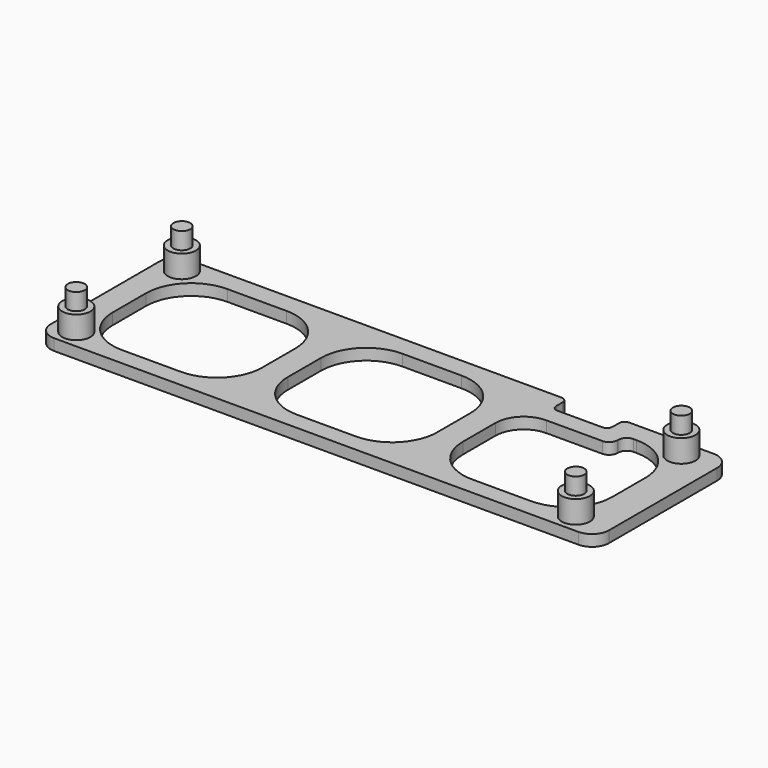
from build123d import *

# Parameters (mm, degrees)
F1_DEPTH = 2
F3_R     = 3
F4_R     = 1
F2_R     = 2.5
F2_R_2   = 1.5
F5_DEPTH = 4
F6_DEPTH = 7


with BuildPart() as f1:
    # F0 (on Top) → F1 (new body)
    with BuildSketch(Plane.XY):
        Polygon((80, -3.433377482), (70, -3.433377482), (70, 0), (0, 0), (0, -30), (99, -30), (99, 0), (80, 0), align=None)
        with BuildLine():
            ThreePointArc((4.5, -11.5), (6.8431457505, -5.8431457505), (12.5, -3.5))
            Line((12.5, -3.5), (23, -3.5))
            ThreePointArc((23, -3.5), (28.6568542495, -5.8431457505), (31, -11.5))
            Line((31, -11.5), (31, -18.9))
            ThreePointArc((31, -18.9), (28.6568542495, -24.5568542495), (23, -26.9))
            Line((23, -26.9), (12.5, -26.9))
            ThreePointArc((12.5, -26.9), (6.8431457505, -24.5568542495), (4.5, -18.9))
            Line((4.5, -18.9), (4.5, -11.5))
        make_face(mode=Mode.SUBTRACT)
        with BuildLine():
            ThreePointArc((35.55, -11.5), (37.8931457505, -5.8431457505), (43.55, -3.5))
            Line((43.55, -3.5), (54.05, -3.5))
            ThreePointArc((54.05, -3.5), (59.7068542495, -5.8431457505), (62.05, -11.5))
            Line((62.05, -11.5), (62.05, -18.9))
            ThreePointArc((62.05, -18.9), (59.7068542495, -24.5568542495), (54.05, -26.9))
            Line((54.05, -26.9), (43.55, -26.9))
            ThreePointArc((43.55, -26.9), (37.8931457505, -24.5568542495), (35.55, -18.9))
            Line((35.55, -18.9), (35.55, -11.5))
        make_face(mode=Mode.SUBTRACT)
        with BuildLine():
            Line((84.5458595753, -3.5), (85.1, -3.5))
            ThreePointArc((85.1, -3.5), (90.7568542495, -5.8431457505), (93.1, -11.5))
            Line((93.1, -11.5), (93.1, -18.9))
            ThreePointArc((93.1, -18.9), (90.7568542495, -24.5568542495), (85.1, -26.9))
            Line((85.1, -26.9), (74.6, -26.9))
            ThreePointArc((74.6, -26.9), (68.9431457505, -24.5568542495), (66.6, -18.9))
            Line((66.6, -18.9), (66.6, -11.6456231289))
            ThreePointArc((66.6, -11.6456231289), (68.0644660941, -8.1100892229), (71.6, -6.6456231289))
            Line((71.6, -6.6456231289), (81.5458595753, -6.6456231289))
            ThreePointArc((81.5458595753, -6.6456231289), (82.6065197471, -6.2062833006), (83.0458595753, -5.1456231289))
            Line((83.0458595753, -5.1456231289), (83.0458595753, -5))
            ThreePointArc((83.0458595753, -5), (83.4851994035, -3.9393398282), (84.5458595753, -3.5))
        make_face(mode=Mode.SUBTRACT)
    extrude(amount=-F1_DEPTH)

    # F3
    f3_edges = [f1.edges().sort_by_distance(p)[0] for p in [
        (0, 0, -1),
        (0, -30, -1),
        (99, -30, -1),
        (99, 0, -1),
    ]]
    fillet(f3_edges, radius=F3_R)

    # F4
    f4_edges = [f1.edges().sort_by_distance(p)[0] for p in [
        (70, -3.433377, -1),
        (80, -3.433377, -1),
        (70, 0, -1),
        (80, 0, -1),
    ]]
    fillet(f4_edges, radius=F4_R)

    # F2 (on face) → F5 (join)
    with BuildSketch(Plane.XY):
        with Locations((4.2, -3.2)):
            Circle(F2_R)
        with Locations((4.2, -3.2)):
            Circle(F2_R_2, mode=Mode.SUBTRACT)
        with Locations((92.8, -3.2)):
            Circle(F2_R)
        with Locations((92.8, -3.2)):
            Circle(F2_R_2, mode=Mode.SUBTRACT)
        with Locations((92.8, -26.6)):
            Circle(F2_R)
        with Locations((92.8, -26.6)):
            Circle(F2_R_2, mode=Mode.SUBTRACT)
        with Locations((4.2, -26.6)):
            Circle(F2_R)
        with Locations((4.2, -26.6)):
            Circle(F2_R_2, mode=Mode.SUBTRACT)
    extrude(amount=F5_DEPTH)

    # F6 (add): faces of the model
    f6_faces = [f1.faces().sort_by_distance(p)[0] for p in [
        (4.2, -3.2, 0),
        (4.2, -26.6, 0),
        (92.8, -3.2, 0),
        (92.8, -26.6, 0),
    ]]
    extrude(f6_faces, amount=F6_DEPTH)


solid = f1.part
